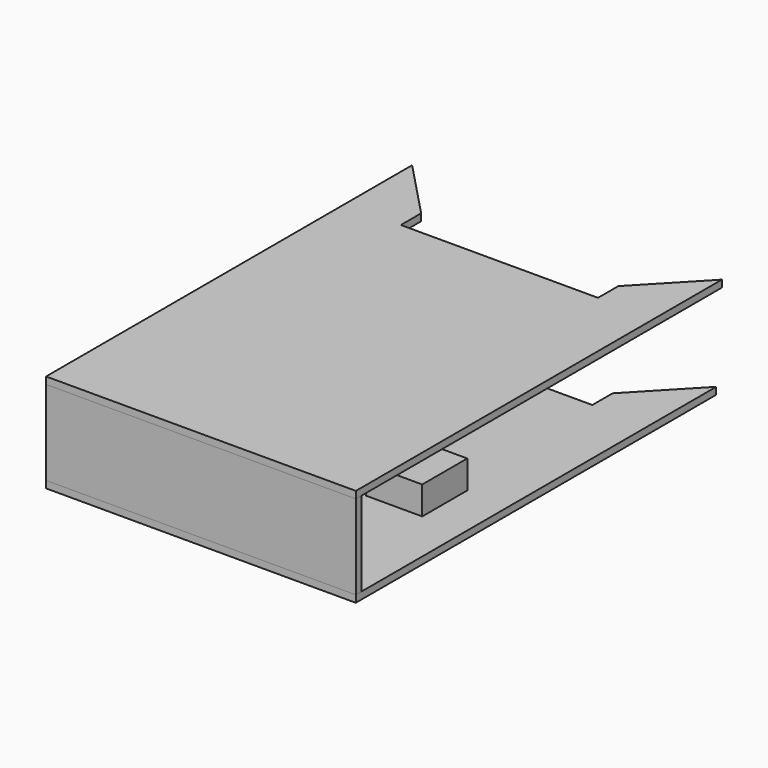
from build123d import *

# Parameters (mm, degrees)
F0_W      = 139.7
F0_H      = 203.2
F1_DEPTH  = 3.175
F3_DEPTH  = 3.175
F4_W      = 25.4
F4_H      = 25.4
F5_DEPTH  = 12.7
F6_W      = 139.7
F6_H      = 3.175
F7_DEPTH  = 38.1
F8_W      = 139.7241105051
F8_H      = 203.2
F9_DEPTH  = 3.175
F11_DEPTH = 25.4
F12_DEPTH = 3.175


# Not quite as in the source:
# - a length typed as a fraction of an inch, garbled in the dataset ("3 / 203.2 mm" for 3/8 in), is restored
# - a feature names something its author has since deleted; it is built from what else it names


with BuildPart() as f1:
    # F0 (on Top) → F1 (new body)
    with BuildSketch(Plane.XY):
        with Locations((15.8455121665, 22.5839115024)):
            Rectangle(F0_W, F0_H)
    extrude(amount=-F1_DEPTH)

    # F2 (on face) → F3 (cut)
    with BuildSketch(Plane.XY):
        Polygon((-28.6044878335, 97.5139115024), (-28.6044878335, 86.0839115024), (60.2955121665, 86.0839115024), (60.2955121665, 97.5139115024), (85.6955121665, 124.1839115024), (-54.0044878335, 124.1839115024), align=None)
    extrude(amount=-F3_DEPTH, mode=Mode.SUBTRACT)

    # F4 (on face) → F5 (join)
    with BuildSketch(Plane.XY):
        with Locations((-22.2290878335, -5.0218783647)):
            Rectangle(F4_W, F4_H)
        with Locations((53.9201121665, -5.0218783647)):
            Rectangle(F4_W, F4_H)
    extrude(amount=F5_DEPTH)


with BuildPart() as f7:
    # F6 (on face) → F7 (new body)
    with BuildSketch(Plane.XY):
        with Locations((15.8455121665, -77.4285884976)):
            Rectangle(F6_W, F6_H)
    extrude(amount=F7_DEPTH)


with BuildPart() as f9:
    # F8 (on face) → F9 (new body)
    with BuildSketch(Plane.XY.offset(38.1)):
        with Locations((15.8575674191, 25.7589115024)):
            Rectangle(F8_W, F8_H)
    extrude(amount=F9_DEPTH)

    # F10 (on face) → F11 (cut)
    with BuildSketch(Plane.XY.offset(41.275)):
        Polygon((-28.6044878335, 100.6889115024), (-28.6044878335, 89.2589115024), (60.3196226716, 89.2589115024), (60.3196226716, 100.6889115024), (85.7196226716, 127.3589115024), (-54.0044878335, 127.3589115024), align=None)
    extrude(amount=-F11_DEPTH, mode=Mode.SUBTRACT)

    # F12 (add): a face of the model
    f12_faces = [f9.faces().sort_by_distance(p)[0] for p in [
        (15.8575674191, -75.8410884976, 39.6875),
    ]]
    extrude(f12_faces, amount=F12_DEPTH)


solid = Compound([f1.part, f7.part, f9.part])
